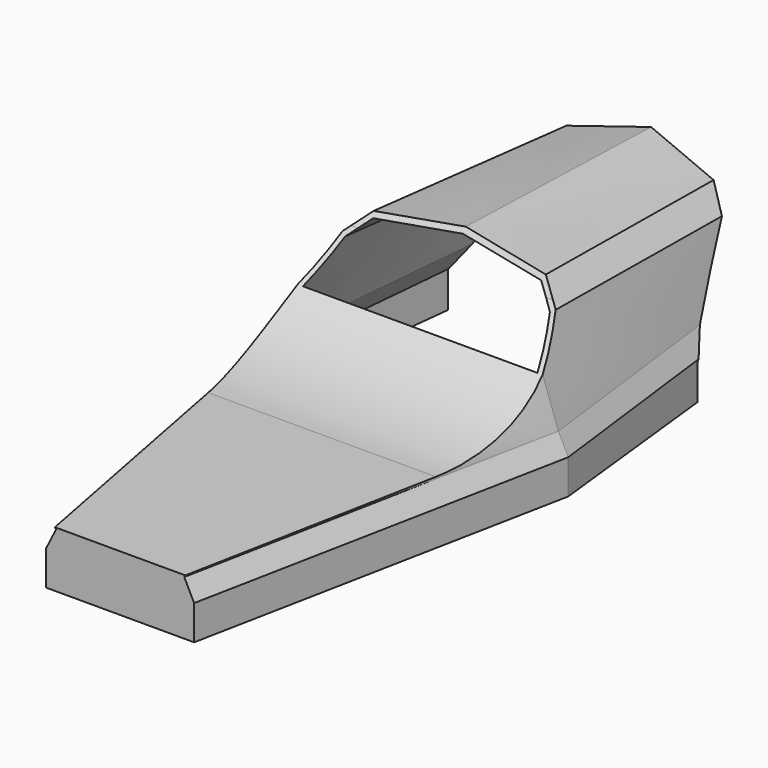
from build123d import *

# Parameters (mm, degrees)
F6_DEPTH  = 150
F11_DEPTH = 150


# Not quite as in the source:
# - a feature names something its author has since deleted; it is built from what else it names


with BuildPart() as f4:
    # F2 (on Front) → F4 section 0
    with BuildSketch(Plane.XZ):
        Polygon((145, 0), (150, 0), (150, 35), (140, 55), (110, 140), (90, 160), (0, 170), (-90, 160), (-110, 140), (-140, 55), (-150, 35), (-150, 0), (-145, 0), (-145, 33.8196601125), (-135.3886514877, 53.0423571371), (-105.6625113622, 137.2664208259), (-87.704664423, 155.2242677651), (0, 164.9692304788), (87.704664423, 155.2242677651), (105.6625113622, 137.2664208259), (135.3886514877, 53.0423571371), (145, 33.8196601125), align=None)
    # F3 (on offset) → F4 section 1
    with BuildSketch(Plane.XZ.offset(-360)):
        Polygon((105, 0), (110, 0), (110, 40), (100, 60), (90, 120), (70, 140), (0, 160), (-70, 140), (-90, 120), (-100, 60), (-110, 40), (-110, 0), (-105, 0), (-105, 38.8196601125), (-95.191631809, 58.4363964945), (-85.3314510321, 117.5974811561), (-67.3806149527, 135.5483172355), (0, 154.7999215077), (67.3806149527, 135.5483172355), (85.3314510321, 117.5974811561), (95.191631809, 58.4363964945), (105, 38.8196601125), align=None)
    loft()

    # F5 (on Right) → F6 (cut, symmetric)
    with BuildSketch(Plane.YZ):
        Polygon((190, 35.5667099357), (190, 0), (189.9669915438, -2.0382583607), (17.2620066122, -21.4886017568), (427.6157569008, -24.6490443013), (429.8257231712, 105.1867231727), (363.7629151344, 190.5601769686), (299.2246747017, 170.2331602573), align=None)
    extrude(amount=F6_DEPTH, both=True, mode=Mode.SUBTRACT)

    # F8 (on Front) → F9 section 0
    with BuildSketch(Plane.XZ):
        Polygon((-150, 0), (150, 0), (150, 35), (140, 55), (110, 140), (90, 160), (0, 170), (-90, 160), (-110, 140), (-140, 55), (-150, 35), align=None)
    # F7 (on offset) → F9 section 1
    with BuildSketch(Plane.XZ.offset(380)):
        Polygon((-75, 0), (75, 0), (75, 35), (65, 55), (110, 130), (90, 150), (0, 160), (-90, 150), (-110, 130), (-65, 55), (-75, 35), align=None)
    loft()

    # F10 (on Right) → F11 (cut, symmetric)
    with BuildSketch(Plane.YZ):
        with BuildLine():
            Line((-388.3555531502, 56.8068251014), (-124.2432887277, 56.8068251014))
            ThreePointArc((-124.2432887277, 56.8068251014), (-31.2629634759, 79.7343565579), (40.3992684554, 143.2602339406))
            Line((40.3992684554, 143.2602339406), (80.7762278766, 201.8068251014))
            Line((80.7762278766, 201.8068251014), (45.3817601157, 256.7874745919))
            Line((45.3817601157, 256.7874745919), (-388.3555531502, 199.957123117))
            Line((-388.3555531502, 199.957123117), (-388.3555531502, 56.8068251014))
        make_face()
    extrude(amount=F11_DEPTH, both=True, mode=Mode.SUBTRACT)


solid = f4.part
